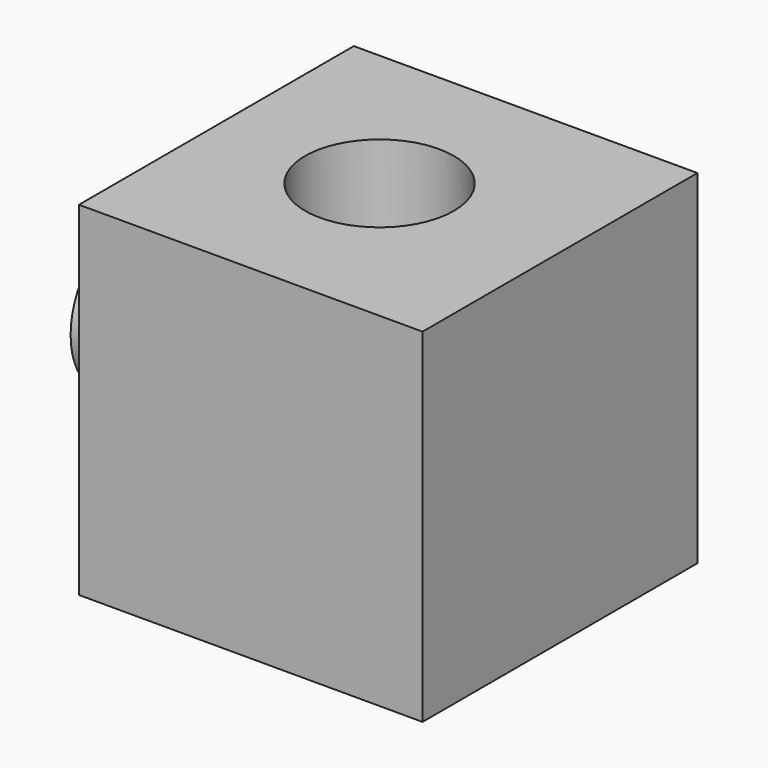
from build123d import *

# Parameters (mm, degrees)
F0_W     = 50.8
F0_H     = 50.8
F1_DEPTH = 50.8
F2_W     = 25.4
F2_H     = 25.4
F4_DEPTH = 12.7
F6_R     = 11
F7_DEPTH = 12.7
F8_R     = 11
F9_DEPTH = 50.8


# Not quite as in the source:
# - a feature names something its author has since deleted; it is built from what else it names


with BuildPart() as f1:
    # F0 (on Front) → F1 (new body)
    with BuildSketch(Plane.XZ):
        with Locations((30.402654475, 1.5070329696)):
            Rectangle(F0_W, F0_H)
    extrude(amount=F1_DEPTH)

    # F6 (on face) → F7 (join)
    with BuildSketch(Plane(origin=(5.002654475, 0, 0), x_dir=(0, -1, 0), z_dir=(-1, 0, 0))):
        with Locations((25.4695527256, 0)):
            Circle(F6_R)
    extrude(amount=F7_DEPTH)

    # F8 (on face) → F9 (cut)
    with BuildSketch(Plane.XY.offset(26.9070329696)):
        with Locations((28.7681911141, -24.9548628926)):
            Circle(F8_R)
    extrude(amount=-F9_DEPTH, mode=Mode.SUBTRACT)


with BuildPart() as f4:
    # F2 (on Front) → F4 (new body)
    with BuildSketch(Plane.XZ):
        with Locations((30.8417927802, 1.382278432)):
            Rectangle(F2_W, F2_H)
    extrude(amount=-F4_DEPTH)


solid = Compound([f1.part, f4.part])
